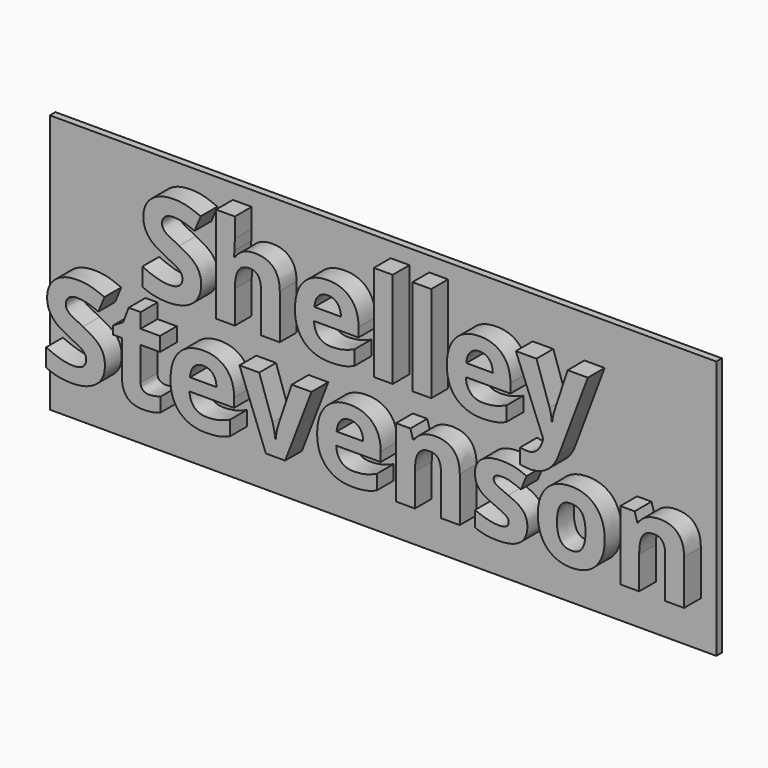
from build123d import *

# Parameters (mm, degrees)
F0_TEXT_SIZE = 18.0555555556
F1_DEPTH     = 3
F2_TEXT_SIZE = 18.0555555556
F3_DEPTH     = 3
F4_W         = 95.162728873
F4_H         = 37
F5_DEPTH     = 1


# Not quite as in the source:
# - Text() gives the source's letters only with a copy of the font that has no kerning and outlines rounded to 1/6400 em; it was checked with that copy


with BuildPart() as f1:
    # F0 (on Front) → F1 (new body)
    with BuildSketch(Plane.XZ):
        with Locations((-32.8032769097, 0)):
            Text('Shelley', F0_TEXT_SIZE, font='Open Sans', font_style=FontStyle.BOLD, text_align=(TextAlign.LEFT, TextAlign.BOTTOM))
    extrude(amount=F1_DEPTH)


with BuildPart() as f3:
    # F2 (on Front) → F3 (new body, through all)
    with BuildSketch(Plane.XZ):
        with Locations((-46.5438368056, -14.6251231368)):
            Text('Stevenson', F2_TEXT_SIZE, font='Open Sans', font_style=FontStyle.BOLD, text_align=(TextAlign.LEFT, TextAlign.BOTTOM))
    extrude(amount=F3_DEPTH)


with BuildPart() as f5:
    # F4 (on Front) → F5 (new body)
    with BuildSketch(Plane.XZ):
        with Locations((0, -2.6531234013)):
            Rectangle(F4_W, F4_H)
    extrude(amount=-F5_DEPTH)


solid = Compound([f1.part, f3.part, f5.part])
